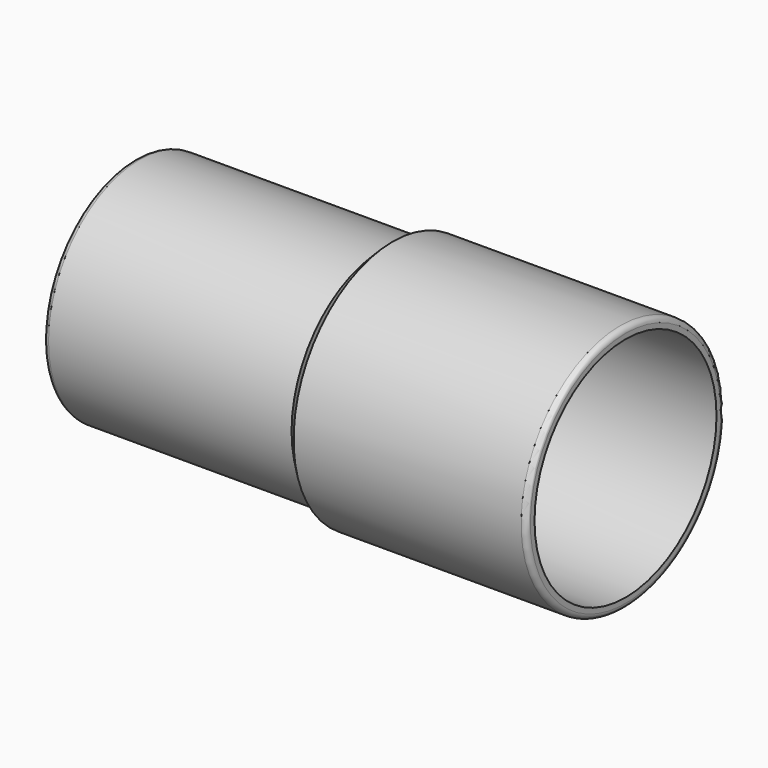
from build123d import *

# Parameters (mm, degrees)
F2_SIZE = 1.99999
F3_R    = 1


# Not quite as in the source:
# - a fillet or chamfer is up to 0.001 mm smaller than in the source, because OpenCascade refuses the exact size


with BuildPart() as f1:
    # F0 (on Front) → F1 (revolve)
    with BuildSketch(Plane.XZ):
        Polygon((-45, 22), (-95, 22), (-95, 20), (-41.2017212381, 20), (-40, 22), (0, 22), (0, 24), (-45, 24), align=None)
    revolve(axis=Axis((-59.3267625081, 0, 0), (-1, 0, 0)))

    # F2 (size 2 in the source; OpenCascade refuses exactly that, so slightly less here)
    f2_edges = [f1.edges().sort_by_distance(p)[0] for p in [
        (-45, 0, -22),
    ]]
    chamfer(f2_edges, length=F2_SIZE)

    # F3
    f3_edges = [f1.edges().sort_by_distance(p)[0] for p in [
        (0, 0, -24),
        (-95, 0, -22),
    ]]
    fillet(f3_edges, radius=F3_R)


solid = f1.part
